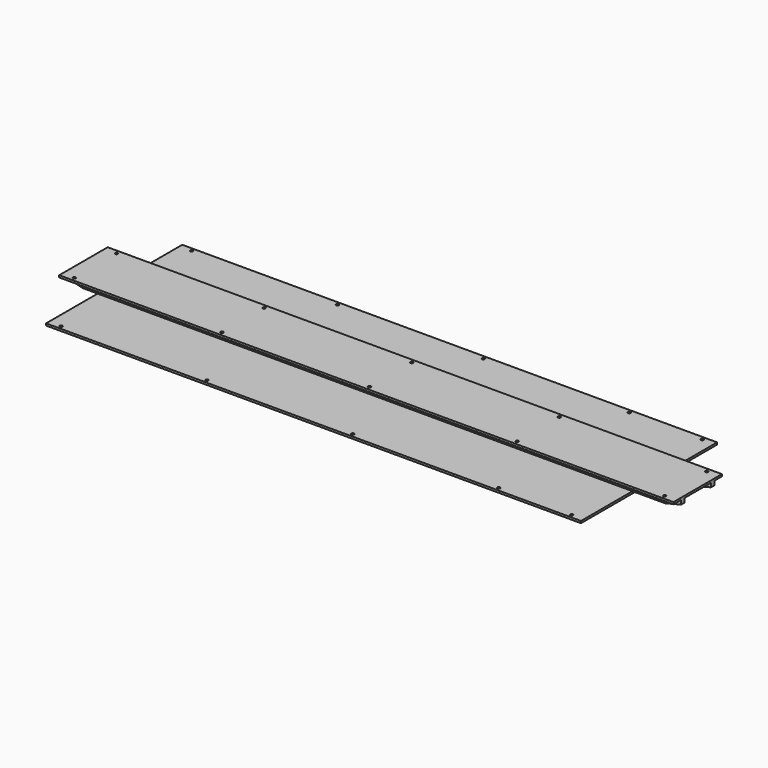
from build123d import *

# Parameters (mm, degrees)
F0_W      = 3352.8
F0_H      = 1066.8
F1_DEPTH  = 12.7
F2_D      = 17.4625
F2_DEPTH  = 50.8
F2_TIP    = 5.2462642799
F4_W      = 3850
F4_H      = 380
F5_DEPTH  = 12.7
F7_D      = 17.4625
F8_W      = 25.4
F8_H      = 50.8
F9_DEPTH  = 3850
F10_SIZE2 = 100
F10_SIZE  = 25
F11_SIZE2 = 100
F11_SIZE  = 25
F12_SIZE2 = 100
F12_SIZE  = 25
F13_SIZE2 = 100
F13_SIZE  = 25


# Not quite as in the source:
# - a length typed as a fraction of an inch, garbled in the dataset ("3 / 203.2 mm" for 3/8 in), is restored


with BuildPart() as f1:
    # F0 (on Top) → F1 (new body)
    with BuildSketch(Plane.XY):
        Rectangle(F0_W, F0_H)
    extrude(amount=F1_DEPTH)

    # F2
    with Locations(Plane(origin=(0, 0, 0), x_dir=(1, 0, 0), z_dir=(0, 0, -1))):
        with Locations((-1600.2, -511.302), (-685.8, -511.302), (228.6, -511.302), (1143, -511.302), (1600.2, -511.302), (1600.2, 511.302), (1143, 511.302), (228.6, 511.302), (-685.8, 511.302), (-1600.2, 511.302)):
            Hole(F2_D / 2, depth=F2_DEPTH)
            with Locations((0, 0, -(F2_DEPTH + F2_TIP / 2))):  # 118° drill point
                Cone(0, F2_D / 2, F2_TIP, mode=Mode.SUBTRACT)



with BuildPart() as f5:
    # F4 (on offset) → F5 (new body)
    with BuildSketch(Plane.XY.offset(76.2)):
        with Locations((56.2, 0)):
            Rectangle(F4_W, F4_H)
    extrude(amount=-F5_DEPTH)

    # F7 (through all)
    with Locations(Plane.XY.offset(76.2)):
        with Locations((-1793.8, 165), (-1793.8, -165), (-868.8, 165), (-868.8, -165), (56.2, 165), (981.2, 165), (56.2, -165), (981.2, -165), (1906.2, 165), (1906.2, -165)):
            Hole(F7_D / 2)


with BuildPart() as f1_1:
    add(f1.part)

    add(f5.part)  # F9 merges F5
    # F8 (on face) → F9 (join)
    with BuildSketch(Plane.YZ.offset(1981.2)):
        with Locations((-117.3, 38.1)):
            Rectangle(F8_W, F8_H)
        with Locations((117.3, 38.1)):
            Rectangle(F8_W, F8_H)
    extrude(amount=-F9_DEPTH)

    # F10
    f10_edges = [f1_1.edges().sort_by_distance(p)[0] for p in [
        (-1868.8, 117.3, 12.7),
    ]]
    f10_side = f1_1.faces().sort_by_distance((-1868.8, 186.147309, 69.85))[0]
    chamfer(f10_edges, length=F10_SIZE, length2=F10_SIZE2, reference=f10_side)

    # F11
    f11_edges = [f1_1.edges().sort_by_distance(p)[0] for p in [
        (-1868.8, -117.3, 12.7),
    ]]
    f11_side = f1_1.faces().sort_by_distance((-1868.8, 126.147309, 50.6))[0]
    chamfer(f11_edges, length=F11_SIZE, length2=F11_SIZE2, reference=f11_side)

    # F12
    f12_edges = [f1_1.edges().sort_by_distance(p)[0] for p in [
        (1981.2, 117.3, 12.7),
    ]]
    f12_side = f1_1.faces().sort_by_distance((1981.2, -186.147309, 69.85))[0]
    chamfer(f12_edges, length=F12_SIZE, length2=F12_SIZE2, reference=f12_side)

    # F13
    f13_edges = [f1_1.edges().sort_by_distance(p)[0] for p in [
        (1981.2, -117.3, 12.7),
    ]]
    f13_side = f1_1.faces().sort_by_distance((1981.2, 108.452691, 50.6))[0]
    chamfer(f13_edges, length=F13_SIZE, length2=F13_SIZE2, reference=f13_side)


solid = f1_1.part
